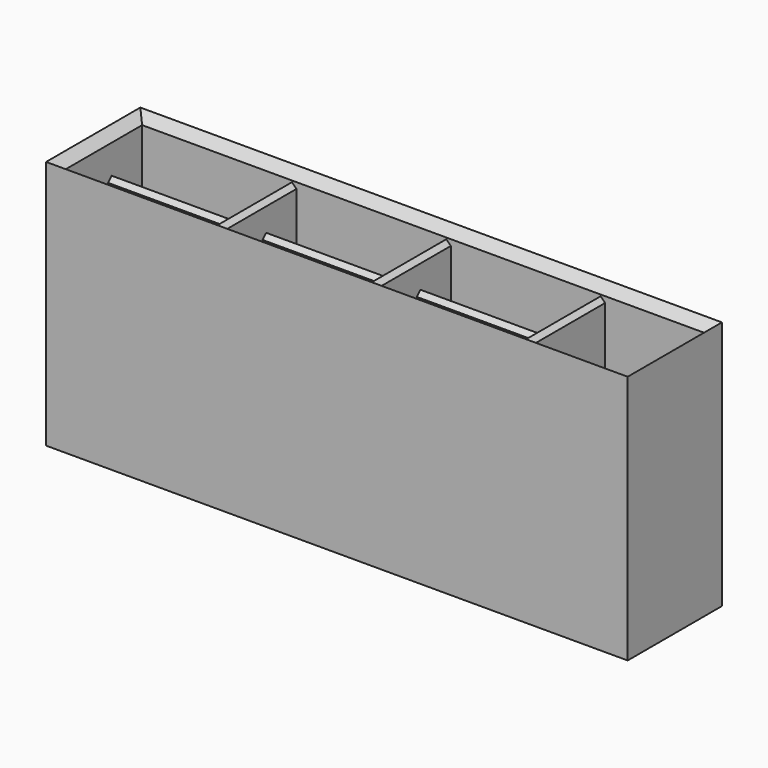
from build123d import *

# Parameters (mm, degrees)
F0_W          = 156
F0_H          = 31.6
F1_DEPTH      = 67
F0_W_2        = 2.4
F0_H_2        = 6
F0_H_3        = 2.4
F0_H_4        = 7
F0_H_5        = 9
F2_DEPTH      = 65.4
F0_W_3        = 39
F3_DEPTH      = 58
F4_DEPTH      = 2.4
F0_W_4        = 27
F5_DEPTH      = 2.4
F6_T1_DEPTH   = 39
F6_T3_DEPTH   = 39
F6_T5_DEPTH   = 39
F6_T7_DEPTH   = 26.8
F6_T12_DEPTH  = 51.3440783422
F6_T17_DEPTH  = 51.3440783422
F6_T22_DEPTH  = 51.3440783422
F6_T27_DEPTH  = 51.3440783422
F6_T32_DEPTH  = 51.3440783422
F6_T37_DEPTH  = 51.3440783422
F6_T42_DEPTH  = 51.3440783422
F6_T47_DEPTH  = 51.3440783422
F6_T52_DEPTH  = 51.3440783422
F6_T57_DEPTH  = 51.3440783422
F6_T62_DEPTH  = 51.3440783422
F6_T67_DEPTH  = 51.3440783422
F6_T72_DEPTH  = 51.3440783422
F6_T77_DEPTH  = 51.3440783422
F6_T82_DEPTH  = 51.3440783422
F6_T87_DEPTH  = 51.3440783422
F6_T92_DEPTH  = 163.5440783422
F6_T98_DEPTH  = 163.5440783422
F6_T104_DEPTH = 39.1440783422
F6_T110_DEPTH = 39.1440783422


# Not quite as in the source:
# - a fillet or chamfer that OpenCascade refuses, or shapes differently, is made with other operations: its cross-section is extruded or revolved along the edge and cut away or added


with BuildPart() as f1:
    # F0 (on Top) → F1 (new body)
    with BuildSketch(Plane.XY):
        Rectangle(F0_W, F0_H)
        Polygon((48.6, 13.4), (75.6, 13.4), (75.6, 4.4), (75.6, 2), (75.6, -5), (75.6, -7.4), (75.6, -13.4), (48.6, -13.4), (46.2, -13.4), (7.2, -13.4), (4.8, -13.4), (-34.2, -13.4), (-36.6, -13.4), (-75.6, -13.4), (-75.6, -7.4), (-75.6, -5), (-75.6, 2), (-75.6, 4.4), (-75.6, 13.4), (-36.6, 13.4), (-34.2, 13.4), (4.8, 13.4), (7.2, 13.4), (46.2, 13.4), align=None, mode=Mode.SUBTRACT)
    extrude(amount=F1_DEPTH)

    # F0 (on Top) → F2 (join)
    with BuildSketch(Plane.XY):
        with Locations((47.4, -10.4)):
            Rectangle(F0_W_2, F0_H_2)
        with Locations((47.4, -6.2)):
            Rectangle(F0_W_2, F0_H_3)
        with Locations((47.4, -1.5)):
            Rectangle(F0_W_2, F0_H_4)
        with Locations((47.4, 3.2)):
            Rectangle(F0_W_2, F0_H_3)
        with Locations((47.4, 8.9)):
            Rectangle(F0_W_2, F0_H_5)
        with Locations((6, 8.9)):
            Rectangle(F0_W_2, F0_H_5)
        with Locations((6, 3.2)):
            Rectangle(F0_W_2, F0_H_3)
        with Locations((6, -1.5)):
            Rectangle(F0_W_2, F0_H_4)
        with Locations((6, -6.2)):
            Rectangle(F0_W_2, F0_H_3)
        with Locations((6, -10.4)):
            Rectangle(F0_W_2, F0_H_2)
        with Locations((-35.4, -10.4)):
            Rectangle(F0_W_2, F0_H_2)
        with Locations((-35.4, -6.2)):
            Rectangle(F0_W_2, F0_H_3)
        with Locations((-35.4, -1.5)):
            Rectangle(F0_W_2, F0_H_4)
        with Locations((-35.4, 3.2)):
            Rectangle(F0_W_2, F0_H_3)
        with Locations((-35.4, 8.9)):
            Rectangle(F0_W_2, F0_H_5)
    extrude(amount=F2_DEPTH)

    # F0 (on Top) → F3 (join)
    with BuildSketch(Plane.XY):
        with Locations((-56.1, -6.2)):
            Rectangle(F0_W_3, F0_H_3)
        with Locations((-56.1, 3.2)):
            Rectangle(F0_W_3, F0_H_3)
        with Locations((-14.7, -6.2)):
            Rectangle(F0_W_3, F0_H_3)
        with Locations((-14.7, 3.2)):
            Rectangle(F0_W_3, F0_H_3)
        with Locations((26.7, 3.2)):
            Rectangle(F0_W_3, F0_H_3)
        with Locations((26.7, -6.2)):
            Rectangle(F0_W_3, F0_H_3)
    extrude(amount=F3_DEPTH)

    # F0 (on Top) → F4 (join)
    with BuildSketch(Plane.XY):
        with Locations((-56.1, -10.4)):
            Rectangle(F0_W_3, F0_H_2)
        with Locations((-56.1, -1.5)):
            Rectangle(F0_W_3, F0_H_4)
        with Locations((-56.1, 8.9)):
            Rectangle(F0_W_3, F0_H_5)
        with Locations((-14.7, 8.9)):
            Rectangle(F0_W_3, F0_H_5)
        with Locations((-14.7, -1.5)):
            Rectangle(F0_W_3, F0_H_4)
        with Locations((-14.7, -10.4)):
            Rectangle(F0_W_3, F0_H_2)
        with Locations((26.7, -10.4)):
            Rectangle(F0_W_3, F0_H_2)
        with Locations((26.7, -1.5)):
            Rectangle(F0_W_3, F0_H_4)
        with Locations((26.7, 8.9)):
            Rectangle(F0_W_3, F0_H_5)
    extrude(amount=F4_DEPTH)

    # F0 (on Top) → F5 (join)
    with BuildSketch(Plane.XY):
        with Locations((62.1, 8.9)):
            Rectangle(F0_W_4, F0_H_5)
        with Locations((62.1, 3.2)):
            Rectangle(F0_W_4, F0_H_3)
        with Locations((62.1, -1.5)):
            Rectangle(F0_W_4, F0_H_4)
        with Locations((62.1, -6.2)):
            Rectangle(F0_W_4, F0_H_3)
        with Locations((62.1, -10.4)):
            Rectangle(F0_W_4, F0_H_2)
    extrude(amount=F5_DEPTH)

    # F6: chamfer of 2.4 on 22 edges, made by hand

    # F6_s2 → F6_t1 (cut)
    with BuildSketch(Plane.YZ.offset(-75.6)):
        Polygon((2, 55.6), (4.4, 58), (2, 58), align=None)
        Polygon((2, 58), (4.4, 55.6), (4.4, 58), align=None)
        Polygon((-7.4, 58), (-5, 55.6), (-5, 58), align=None)
        Polygon((-7.4, 55.6), (-5, 58), (-7.4, 58), align=None)
    extrude(amount=F6_T1_DEPTH, mode=Mode.SUBTRACT)

    # F6_s4 → F6_t3 (cut)
    with BuildSketch(Plane.YZ.offset(-34.2)):
        Polygon((-7.4, 55.6), (-5, 58), (-7.4, 58), align=None)
        Polygon((-7.4, 58), (-5, 55.6), (-5, 58), align=None)
        Polygon((2, 58), (4.4, 55.6), (4.4, 58), align=None)
        Polygon((2, 55.6), (4.4, 58), (2, 58), align=None)
    extrude(amount=F6_T3_DEPTH, mode=Mode.SUBTRACT)

    # F6_s6 → F6_t5 (cut)
    with BuildSketch(Plane.YZ.offset(7.2)):
        Polygon((2, 55.6), (4.4, 58), (2, 58), align=None)
        Polygon((2, 58), (4.4, 55.6), (4.4, 58), align=None)
        Polygon((-7.4, 55.6), (-5, 58), (-7.4, 58), align=None)
        Polygon((-7.4, 58), (-5, 55.6), (-5, 58), align=None)
    extrude(amount=F6_T5_DEPTH, mode=Mode.SUBTRACT)

    # F6_s8 → F6_t7 (cut)
    with BuildSketch(Plane.XZ.offset(-13.4)):
        Polygon((-36.6, 63), (-34.2, 65.4), (-36.6, 65.4), align=None)
        Polygon((-36.6, 65.4), (-34.2, 63), (-34.2, 65.4), align=None)
        Polygon((4.8, 63), (7.2, 65.4), (4.8, 65.4), align=None)
        Polygon((4.8, 65.4), (7.2, 63), (7.2, 65.4), align=None)
        Polygon((46.2, 63), (48.6, 65.4), (46.2, 65.4), align=None)
        Polygon((46.2, 65.4), (48.6, 63), (48.6, 65.4), align=None)
    extrude(amount=F6_T7_DEPTH, mode=Mode.SUBTRACT)


with BuildPart() as f6_tool10:
    # F6_s11 → F6_t12 (new body)
    with BuildSketch(Plane.YZ.offset(-81.7720391711)):
        Polygon((2, 55.6), (4.4, 58), (2, 58), align=None)
    extrude(amount=F6_T12_DEPTH)

    split(bisect_by=Plane.YZ.offset(-34.2), keep=Keep.TOP)


with BuildPart() as f1_1:
    add(f1.part)

    # F6_t9: cut F6_tool10
    add(f6_tool10.part, mode=Mode.SUBTRACT)


with BuildPart() as f6_tool15:
    # F6_s16 → F6_t17 (new body)
    with BuildSketch(Plane.YZ.offset(-30.4279608289)):
        Polygon((2, 58), (4.4, 55.6), (4.4, 58), align=None)
    extrude(amount=-F6_T17_DEPTH)

    split(bisect_by=Plane.YZ.offset(-34.2), keep=Keep.TOP)


with BuildPart() as f1_2:
    add(f1_1.part)

    # F6_t14: cut F6_tool15
    add(f6_tool15.part, mode=Mode.SUBTRACT)


with BuildPart() as f6_tool20:
    # F6_s21 → F6_t22 (new body)
    with BuildSketch(Plane.YZ.offset(-30.4279608289)):
        Polygon((-7.4, 58), (-5, 55.6), (-5, 58), align=None)
    extrude(amount=-F6_T22_DEPTH)

    split(bisect_by=Plane.YZ.offset(-34.2), keep=Keep.TOP)


with BuildPart() as f1_3:
    add(f1_2.part)

    # F6_t19: cut F6_tool20
    add(f6_tool20.part, mode=Mode.SUBTRACT)


with BuildPart() as f6_tool25:
    # F6_s26 → F6_t27 (new body)
    with BuildSketch(Plane.YZ.offset(-81.7720391711)):
        Polygon((-7.4, 55.6), (-5, 58), (-7.4, 58), align=None)
    extrude(amount=F6_T27_DEPTH)

    split(bisect_by=Plane.YZ.offset(-34.2), keep=Keep.TOP)


with BuildPart() as f1_4:
    add(f1_3.part)

    # F6_t24: cut F6_tool25
    add(f6_tool25.part, mode=Mode.SUBTRACT)


with BuildPart() as f6_tool30:
    # F6_s31 → F6_t32 (new body)
    with BuildSketch(Plane.YZ.offset(-40.3720391711)):
        Polygon((-7.4, 55.6), (-5, 58), (-7.4, 58), align=None)
    extrude(amount=F6_T32_DEPTH)

    split(bisect_by=Plane.YZ.offset(-36.6), keep=Keep.BOTTOM)


with BuildPart() as f1_5:
    add(f1_4.part)

    # F6_t29: cut F6_tool30
    add(f6_tool30.part, mode=Mode.SUBTRACT)


with BuildPart() as f6_tool35:
    # F6_s36 → F6_t37 (new body)
    with BuildSketch(Plane.YZ.offset(-40.3720391711)):
        Polygon((-7.4, 55.6), (-5, 58), (-7.4, 58), align=None)
    extrude(amount=F6_T37_DEPTH)

    split(bisect_by=Plane.YZ.offset(7.2), keep=Keep.TOP)


with BuildPart() as f1_6:
    add(f1_5.part)

    # F6_t34: cut F6_tool35
    add(f6_tool35.part, mode=Mode.SUBTRACT)


with BuildPart() as f6_tool40:
    # F6_s41 → F6_t42 (new body)
    with BuildSketch(Plane.YZ.offset(10.9720391711)):
        Polygon((-7.4, 58), (-5, 55.6), (-5, 58), align=None)
    extrude(amount=-F6_T42_DEPTH)

    split(bisect_by=Plane.YZ.offset(7.2), keep=Keep.TOP)


with BuildPart() as f1_7:
    add(f1_6.part)

    # F6_t39: cut F6_tool40
    add(f6_tool40.part, mode=Mode.SUBTRACT)


with BuildPart() as f6_tool45:
    # F6_s46 → F6_t47 (new body)
    with BuildSketch(Plane.YZ.offset(10.9720391711)):
        Polygon((-7.4, 58), (-5, 55.6), (-5, 58), align=None)
    extrude(amount=-F6_T47_DEPTH)

    split(bisect_by=Plane.YZ.offset(-36.6), keep=Keep.BOTTOM)


with BuildPart() as f1_8:
    add(f1_7.part)

    # F6_t44: cut F6_tool45
    add(f6_tool45.part, mode=Mode.SUBTRACT)


with BuildPart() as f6_tool50:
    # F6_s51 → F6_t52 (new body)
    with BuildSketch(Plane.YZ.offset(10.9720391711)):
        Polygon((2, 58), (4.4, 55.6), (4.4, 58), align=None)
    extrude(amount=-F6_T52_DEPTH)

    split(bisect_by=Plane.YZ.offset(7.2), keep=Keep.TOP)


with BuildPart() as f1_9:
    add(f1_8.part)

    # F6_t49: cut F6_tool50
    add(f6_tool50.part, mode=Mode.SUBTRACT)


with BuildPart() as f6_tool55:
    # F6_s56 → F6_t57 (new body)
    with BuildSketch(Plane.YZ.offset(10.9720391711)):
        Polygon((2, 58), (4.4, 55.6), (4.4, 58), align=None)
    extrude(amount=-F6_T57_DEPTH)

    split(bisect_by=Plane.YZ.offset(-36.6), keep=Keep.BOTTOM)


with BuildPart() as f1_10:
    add(f1_9.part)

    # F6_t54: cut F6_tool55
    add(f6_tool55.part, mode=Mode.SUBTRACT)


with BuildPart() as f6_tool60:
    # F6_s61 → F6_t62 (new body)
    with BuildSketch(Plane.YZ.offset(-40.3720391711)):
        Polygon((2, 55.6), (4.4, 58), (2, 58), align=None)
    extrude(amount=F6_T62_DEPTH)

    split(bisect_by=Plane.YZ.offset(-36.6), keep=Keep.BOTTOM)


with BuildPart() as f1_11:
    add(f1_10.part)

    # F6_t59: cut F6_tool60
    add(f6_tool60.part, mode=Mode.SUBTRACT)


with BuildPart() as f6_tool65:
    # F6_s66 → F6_t67 (new body)
    with BuildSketch(Plane.YZ.offset(-40.3720391711)):
        Polygon((2, 55.6), (4.4, 58), (2, 58), align=None)
    extrude(amount=F6_T67_DEPTH)

    split(bisect_by=Plane.YZ.offset(7.2), keep=Keep.TOP)


with BuildPart() as f1_12:
    add(f1_11.part)

    # F6_t64: cut F6_tool65
    add(f6_tool65.part, mode=Mode.SUBTRACT)


with BuildPart() as f6_tool70:
    # F6_s71 → F6_t72 (new body)
    with BuildSketch(Plane.YZ.offset(1.0279608289)):
        Polygon((2, 55.6), (4.4, 58), (2, 58), align=None)
    extrude(amount=F6_T72_DEPTH)

    split(bisect_by=Plane.YZ.offset(4.8), keep=Keep.BOTTOM)


with BuildPart() as f1_13:
    add(f1_12.part)

    # F6_t69: cut F6_tool70
    add(f6_tool70.part, mode=Mode.SUBTRACT)


with BuildPart() as f6_tool75:
    # F6_s76 → F6_t77 (new body)
    with BuildSketch(Plane.YZ.offset(52.3720391711)):
        Polygon((2, 58), (4.4, 55.6), (4.4, 58), align=None)
    extrude(amount=-F6_T77_DEPTH)

    split(bisect_by=Plane.YZ.offset(4.8), keep=Keep.BOTTOM)


with BuildPart() as f1_14:
    add(f1_13.part)

    # F6_t74: cut F6_tool75
    add(f6_tool75.part, mode=Mode.SUBTRACT)


with BuildPart() as f6_tool80:
    # F6_s81 → F6_t82 (new body)
    with BuildSketch(Plane.YZ.offset(1.0279608289)):
        Polygon((-7.4, 55.6), (-5, 58), (-7.4, 58), align=None)
    extrude(amount=F6_T82_DEPTH)

    split(bisect_by=Plane.YZ.offset(4.8), keep=Keep.BOTTOM)


with BuildPart() as f1_15:
    add(f1_14.part)

    # F6_t79: cut F6_tool80
    add(f6_tool80.part, mode=Mode.SUBTRACT)


with BuildPart() as f6_tool85:
    # F6_s86 → F6_t87 (new body)
    with BuildSketch(Plane.YZ.offset(52.3720391711)):
        Polygon((-7.4, 58), (-5, 55.6), (-5, 58), align=None)
    extrude(amount=-F6_T87_DEPTH)

    split(bisect_by=Plane.YZ.offset(4.8), keep=Keep.BOTTOM)


with BuildPart() as f1_16:
    add(f1_15.part)

    # F6_t84: cut F6_tool85
    add(f6_tool85.part, mode=Mode.SUBTRACT)


with BuildPart() as f6_tool90:
    # F6_s91 → F6_t92 (new body)
    with BuildSketch(Plane.YZ.offset(81.7720391711)):
        Polygon((15.8, 67), (13.4, 64.6), (13.4, 67), align=None)
    extrude(amount=-F6_T92_DEPTH)

    split(bisect_by=Plane(origin=(5.5, 0, -5.5), x_dir=(0, 1, 0), z_dir=(-0.7071067812, 0, 0.7071067812)), keep=Keep.TOP)

    split(bisect_by=Plane(origin=(-5.5, 0, -5.5), x_dir=(0, 1, 0), z_dir=(0.7071067812, 0, 0.7071067812)), keep=Keep.TOP)


with BuildPart() as f1_17:
    add(f1_16.part)

    # F6_t89: cut F6_tool90
    add(f6_tool90.part, mode=Mode.SUBTRACT)


with BuildPart() as f6_tool96:
    # F6_s97 → F6_t98 (new body)
    with BuildSketch(Plane.YZ.offset(-81.7720391711)):
        Polygon((-15.8, 67), (-13.4, 64.6), (-13.4, 67), align=None)
    extrude(amount=F6_T98_DEPTH)

    split(bisect_by=Plane(origin=(5.5, 0, -5.5), x_dir=(0, 1, 0), z_dir=(-0.7071067812, 0, 0.7071067812)), keep=Keep.TOP)

    split(bisect_by=Plane(origin=(-5.5, 0, -5.5), x_dir=(0, 1, 0), z_dir=(0.7071067812, 0, 0.7071067812)), keep=Keep.TOP)


with BuildPart() as f1_18:
    add(f1_17.part)

    # F6_t95: cut F6_tool96
    add(f6_tool96.part, mode=Mode.SUBTRACT)


with BuildPart() as f6_tool102:
    # F6_s103 → F6_t104 (new body)
    with BuildSketch(Plane.XZ.offset(-19.5720391711)):
        Polygon((-78, 67), (-75.6, 64.6), (-75.6, 67), align=None)
    extrude(amount=F6_T104_DEPTH)

    split(bisect_by=Plane(origin=(0, -25.6, 25.6), x_dir=(1, 0, 0), z_dir=(0, -0.7071067812, 0.7071067812)), keep=Keep.TOP)

    split(bisect_by=Plane(origin=(0, 25.6, 25.6), x_dir=(1, 0, 0), z_dir=(0, 0.7071067812, 0.7071067812)), keep=Keep.TOP)


with BuildPart() as f1_19:
    add(f1_18.part)

    # F6_t101: cut F6_tool102
    add(f6_tool102.part, mode=Mode.SUBTRACT)


with BuildPart() as f6_tool108:
    # F6_s109 → F6_t110 (new body)
    with BuildSketch(Plane.XZ.offset(19.5720391711)):
        Polygon((78, 67), (75.6, 64.6), (75.6, 67), align=None)
    extrude(amount=-F6_T110_DEPTH)

    split(bisect_by=Plane(origin=(0, -25.6, 25.6), x_dir=(1, 0, 0), z_dir=(0, -0.7071067812, 0.7071067812)), keep=Keep.TOP)

    split(bisect_by=Plane(origin=(0, 25.6, 25.6), x_dir=(1, 0, 0), z_dir=(0, 0.7071067812, 0.7071067812)), keep=Keep.TOP)


with BuildPart() as f1_20:
    add(f1_19.part)

    # F6_t107: cut F6_tool108
    add(f6_tool108.part, mode=Mode.SUBTRACT)


solid = f1_20.part
